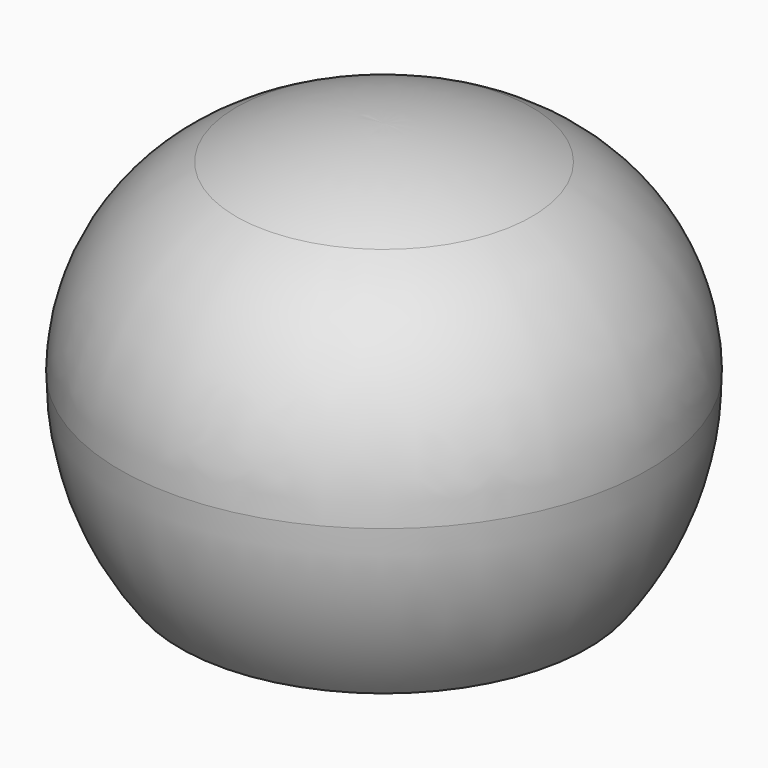
from build123d import *

# Parameters (mm, degrees)
F2_R = 1.2
F3_R = 1.5


# Not quite as in the source:
# - ends of sketch curves that miss each other by under 0.0002 mm in the source are joined


with BuildPart() as f1:
    # F0 (on Front) → F1 (revolve)
    with BuildSketch(Plane.XZ):
        with BuildLine():
            ThreePointArc((-3.15, 22.237062203), (-3.9031761874, 22.0947631243), (-4.65, 21.92220128))
            Line((-4.65, 21.92220128), (-4.65, 17.737062203))
            Line((-4.65, 17.737062203), (-3.15, 17.737062203))
            Line((-3.15, 17.737062203), (-3.15, 22.237062203))
        make_face()
        with BuildLine():
            ThreePointArc((-8.3124990512, 20.5851502634), (-6.5156367124, 21.3478704117), (-4.65, 21.92220128))
            ThreePointArc((-4.65, 21.92220128), (-3.9031761874, 22.0947631243), (-3.15, 22.237062203))
            ThreePointArc((-3.15, 22.237062203), (-1.5804774821, 22.4341514446), (0, 22.5))
            Line((0, 22.5), (0, 24))
            ThreePointArc((0, 24), (-4.6018178135, 23.4768187956), (-8.9687491511, 21.933978275))
            ThreePointArc((-8.9687491511, 21.933978275), (-14.0973903538, 17.3228740591), (-16, 10.6937474793))
            ThreePointArc((-16, 10.6937474793), (-15.0630616225, 5.0444120813), (-12.3525726045, 0))
            Line((-12.3525726045, 0), (-10.4014182071, 0))
            ThreePointArc((-10.4014182071, 0), (-13.4402589307, 4.9676099375), (-14.4999996005, 10.6937474793))
            ThreePointArc((-14.4999996005, 10.6937474793), (-12.8257031653, 16.5273786831), (-8.3124990512, 20.5851502634))
        make_face()
    revolve(axis=Axis((0, 0, 23.25), (0, 0, 1)))

    # F2
    f2_edges = [f1.edges().sort_by_distance(p)[0] for p in [
        (3.15, 0, 17.737062),
    ]]
    fillet(f2_edges, radius=F2_R)

    # F3
    f3_edges = [f1.edges().sort_by_distance(p)[0] for p in [
        (4.65, 0, 21.922201),
    ]]
    fillet(f3_edges, radius=F3_R)


solid = f1.part
